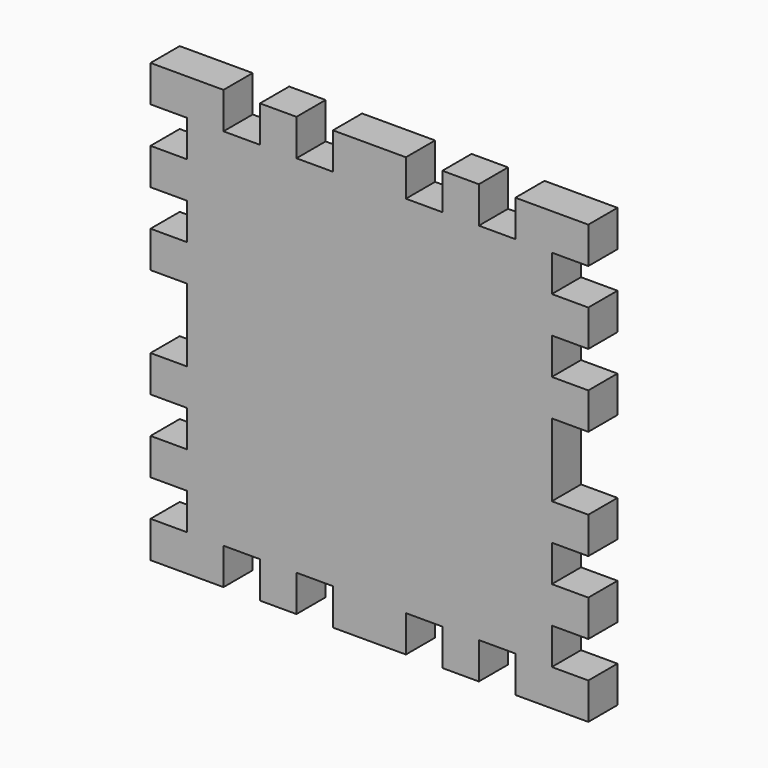
from build123d import *

# Parameters (mm, degrees)
F0_W     = 76.2
F0_H     = 76.2
F1_DEPTH = 6.35
F2_W     = 6.35
F2_H     = 6.35
F3_DEPTH = 6.351
F4_W     = 6.35
F4_H     = 6.35
F5_DEPTH = 6.351
F6_W     = 6.35
F6_H     = 6.35
F6_H_2   = 12.7
F7_DEPTH = 6.351


# Not quite as in the source:
# - a feature names something its author has since deleted; it is built from what else it names


with BuildPart() as f1:
    # F0 (on Front) → F1 (new body)
    with BuildSketch(Plane.XZ):
        Rectangle(F0_W, F0_H)
    extrude(amount=F1_DEPTH)

    # F2 (on face) → F3 (cut, through all)
    with BuildSketch(Plane.XZ.offset(6.35)):
        with Locations((-22.225, 34.925)):
            Rectangle(F2_W, F2_H)
        with Locations((-9.525, 34.925)):
            Rectangle(F2_W, F2_H)
        with Locations((9.525, 34.925)):
            Rectangle(F2_W, F2_H)
        with Locations((22.225, 34.925)):
            Rectangle(F2_W, F2_H)
    extrude(amount=-F3_DEPTH, mode=Mode.SUBTRACT)

    # F4 (on face) → F5 (cut, through all)
    with BuildSketch(Plane.XZ.offset(6.35)):
        with Locations((-9.525, -34.925)):
            Rectangle(F4_W, F4_H)
        with Locations((9.525, -34.925)):
            Rectangle(F4_W, F4_H)
        with Locations((22.225, -34.925)):
            Rectangle(F4_W, F4_H)
        with Locations((-22.225, -34.925)):
            Rectangle(F4_W, F4_H)
    extrude(amount=-F5_DEPTH, mode=Mode.SUBTRACT)

    # F6 (on face) → F7 (cut, through all)
    with BuildSketch(Plane.XZ.offset(6.35)):
        with Locations((-34.925, -28.575)):
            Rectangle(F6_W, F6_H)
        with Locations((-34.925, -15.875)):
            Rectangle(F6_W, F6_H)
        with Locations((-34.925, 0)):
            Rectangle(F6_W, F6_H_2)
        with Locations((-34.925, 15.875)):
            Rectangle(F6_W, F6_H)
        with Locations((-34.925, 28.575)):
            Rectangle(F6_W, F6_H)
        with Locations((34.925, -28.575)):
            Rectangle(F6_W, F6_H)
        with Locations((34.925, -15.875)):
            Rectangle(F6_W, F6_H)
        with Locations((34.925, -3.175)):
            Rectangle(F6_W, F6_H)
        with Locations((34.925, 3.175)):
            Rectangle(F6_W, F6_H)
        with Locations((34.925, 15.875)):
            Rectangle(F6_W, F6_H)
        with Locations((34.925, 28.575)):
            Rectangle(F6_W, F6_H)
    extrude(amount=-F7_DEPTH, mode=Mode.SUBTRACT)


solid = f1.part
